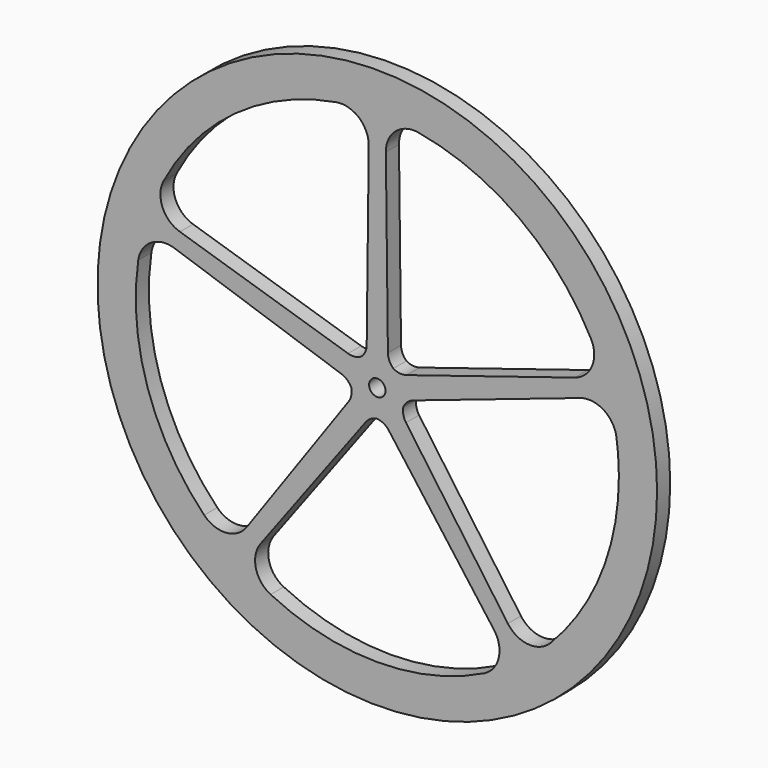
from build123d import *

# Parameters (mm, degrees)
F0_R        = 51.2
F1_DEPTH    = 1.5
F2_T1_DEPTH = 3
F3_R        = 5.08


# Not quite as in the source:
# - a fillet or chamfer that OpenCascade refuses, or shapes differently, is made with other operations: its cross-section is extruded or revolved along the edge and cut away or added


with BuildPart() as f1:
    # F0 (on Front) → F1 (new body, symmetric)
    with BuildSketch(Plane.XZ):
        Circle(F0_R)
        with BuildLine():
            ThreePointArc((1.5, 44.1745401787), (25.9801081513, 35.7585511514), (41.5489587997, 15.0772684084))
            ThreePointArc((41.5489587997, 15.0772684084), (42.0366980202, 13.6585511514), (42.4760097829, 12.2240988595))
            ThreePointArc((42.4760097829, 12.2240988595), (43.7668803572, 6.1725346333), (44.2, 0))
            ThreePointArc((44.2, 0), (39.7173586616, -19.3951391062), (27.1786687354, -34.8562758448))
            ThreePointArc((27.1786687354, -34.8562758448), (25.9801081513, -35.7585511514), (24.7516177523, -36.6196316017))
            ThreePointArc((24.7516177523, -36.6196316017), (0, -44.2), (-24.7516177523, -36.6196316017))
            ThreePointArc((-24.7516177523, -36.6196316017), (-25.9801081513, -35.7585511514), (-27.1786687354, -34.8562758448))
            ThreePointArc((-27.1786687354, -34.8562758448), (-42.0366980202, -13.6585511514), (-42.4760097829, 12.2240988595))
            ThreePointArc((-42.4760097829, 12.2240988595), (-42.0366980202, 13.6585511514), (-41.5489587997, 15.0772684084))
            ThreePointArc((-41.5489587997, 15.0772684084), (-25.9801081513, 35.7585511514), (-1.5, 44.1745401787))
            ThreePointArc((-1.5, 44.1745401787), (0, 44.2), (1.5, 44.1745401787))
        make_face(mode=Mode.SUBTRACT)
        with BuildLine():
            Line((-24.7516177523, -36.6196316017), (-1.118469097, -4.8732973313))
            ThreePointArc((-1.118469097, -4.8732973313), (-2.9389262615, -4.0450849719), (-4.2891552241, -2.569659017))
            Line((-4.2891552241, -2.569659017), (-27.1786687354, -34.8562758448))
            ThreePointArc((-27.1786687354, -34.8562758448), (-25.9801081513, -35.7585511514), (-24.7516177523, -36.6196316017))
        make_face()
        with BuildLine():
            ThreePointArc((-4.9804071414, -0.4422043711), (-4.7552825815, 1.5450849719), (-3.7693128085, 3.2851607193))
            Line((-3.7693128085, 3.2851607193), (-41.5489587997, 15.0772684084))
            ThreePointArc((-41.5489587997, 15.0772684084), (-42.0366980202, 13.6585511514), (-42.4760097829, 12.2240988595))
            Line((-42.4760097829, 12.2240988595), (-4.9804071414, -0.4422043711))
        make_face()
        with BuildLine():
            ThreePointArc((-1.9595917942, 4.6), (0, 5), (1.9595917942, 4.6))
            Line((1.9595917942, 4.6), (1.5, 44.1745401787))
            ThreePointArc((1.5, 44.1745401787), (0, 44.2), (-1.5, 44.1745401787))
            Line((-1.5, 44.1745401787), (-1.9595917942, 4.6))
        make_face()
        with BuildLine():
            ThreePointArc((3.7693128085, 3.2851607193), (4.6822304537, 1.7540575757), (5, 0))
            ThreePointArc((5, 0), (4.9950993837, -0.2213191055), (4.9804071414, -0.4422043711))
            Line((4.9804071414, -0.4422043711), (42.4760097829, 12.2240988595))
            ThreePointArc((42.4760097829, 12.2240988595), (42.0366980202, 13.6585511514), (41.5489587997, 15.0772684084))
            Line((41.5489587997, 15.0772684084), (3.7693128085, 3.2851607193))
        make_face()
        with BuildLine():
            Line((27.1786687354, -34.8562758448), (4.2891552241, -2.569659017))
            ThreePointArc((4.2891552241, -2.569659017), (2.9389262615, -4.0450849719), (1.118469097, -4.8732973313))
            Line((1.118469097, -4.8732973313), (24.7516177523, -36.6196316017))
            ThreePointArc((24.7516177523, -36.6196316017), (25.9801081513, -35.7585511514), (27.1786687354, -34.8562758448))
        make_face()
        with BuildLine():
            ThreePointArc((4.9804071414, -0.4422043711), (4.9950993837, -0.2213191055), (5, 0))
            ThreePointArc((5, 0), (4.6822304537, 1.7540575757), (3.7693128085, 3.2851607193))
            ThreePointArc((3.7693128085, 3.2851607193), (2.9389262615, 4.0450849719), (1.9595917942, 4.6))
            ThreePointArc((1.9595917942, 4.6), (0, 5), (-1.9595917942, 4.6))
            ThreePointArc((-1.9595917942, 4.6), (-2.9389262615, 4.0450849719), (-3.7693128085, 3.2851607193))
            ThreePointArc((-3.7693128085, 3.2851607193), (-4.7552825815, 1.5450849719), (-4.9804071414, -0.4422043711))
            ThreePointArc((-4.9804071414, -0.4422043711), (-4.7552825815, -1.5450849719), (-4.2891552241, -2.569659017))
            ThreePointArc((-4.2891552241, -2.569659017), (-2.9389262615, -4.0450849719), (-1.118469097, -4.8732973313))
            ThreePointArc((-1.118469097, -4.8732973313), (0, -5), (1.118469097, -4.8732973313))
            ThreePointArc((1.118469097, -4.8732973313), (2.9389262615, -4.0450849719), (4.2891552241, -2.569659017))
            ThreePointArc((4.2891552241, -2.569659017), (4.7552825815, -1.5450849719), (4.9804071414, -0.4422043711))
        make_face()
        with BuildLine():
            ThreePointArc((0, 1.5), (1.0606601718, 1.0606601718), (1.5, 0))
            ThreePointArc((1.5, 0), (-1.0606601718, -1.0606601718), (0, 1.5))
        make_face(mode=Mode.SUBTRACT)
    extrude(amount=F1_DEPTH, both=True)

    # F2: fillet of radius 3 on 10 edges, made by hand

    # F2_s2 → F2_t1 (join)
    with BuildSketch(Plane.XZ.offset(-1.5)):
        with BuildLine():
            ThreePointArc((3.0875868977, 3.9327861815), (2.2498717307, 4.9648804635), (1.9403413197, 6.2576202799))
            Line((1.9403413197, 6.2576202799), (1.9595917942, 4.6))
            ThreePointArc((1.9595917942, 4.6), (2.5455444913, 4.303510572), (3.0875868977, 3.9327861815))
        make_face()
        with BuildLine():
            ThreePointArc((2.7861851021, 4.151767404), (4.0266333175, 3.6739876086), (5.351752101, 3.7790852667))
            Line((5.351752101, 3.7790852667), (3.7693128085, 3.2851607193))
            ThreePointArc((3.7693128085, 3.2851607193), (3.3062652647, 3.7508145781), (2.7861851021, 4.151767404))
        make_face()
        with BuildLine():
            ThreePointArc((-2.7861851021, 4.151767404), (-4.0266333175, 3.6739876086), (-5.351752101, 3.7790852667))
            Line((-5.351752101, 3.7790852667), (-3.7693128085, 3.2851607193))
            ThreePointArc((-3.7693128085, 3.2851607193), (-3.3062652647, 3.7508145781), (-2.7861851021, 4.151767404))
        make_face()
        with BuildLine():
            ThreePointArc((-3.0875868977, 3.9327861815), (-2.2498717307, 4.9648804635), (-1.9403413197, 6.2576202799))
            Line((-1.9403413197, 6.2576202799), (-1.9595917942, 4.6))
            ThreePointArc((-1.9595917942, 4.6), (-2.5455444913, 4.303510572), (-3.0875868977, 3.9327861815))
        make_face()
        with BuildLine():
            ThreePointArc((-4.6944187481, -1.7211718734), (-5.4171305174, -0.605522732), (-6.5509489863, 0.0883367549))
            Line((-6.5509489863, 0.0883367549), (-4.9804071414, -0.4422043711))
            ThreePointArc((-4.9804071414, -0.4422043711), (-4.8794982801, -1.0910987737), (-4.6944187481, -1.7211718734))
        make_face()
        with BuildLine():
            ThreePointArc((-4.8095439897, -1.3668528124), (-4.7384679811, -2.6942312472), (-5.2479060175, -3.9220171386))
            Line((-5.2479060175, -3.9220171386), (-4.2891552241, -2.569659017))
            ThreePointArc((-4.2891552241, -2.569659017), (-4.5889288007, -1.9853796772), (-4.8095439897, -1.3668528124))
        make_face()
        with BuildLine():
            ThreePointArc((4.6944187481, -1.7211718734), (5.4171305174, -0.605522732), (6.5509489863, 0.0883367549))
            Line((6.5509489863, 0.0883367549), (4.9804071414, -0.4422043711))
            ThreePointArc((4.9804071414, -0.4422043711), (4.8794982801, -1.0910987737), (4.6944187481, -1.7211718734))
        make_face()
        with BuildLine():
            ThreePointArc((4.8095439897, -1.3668528124), (4.7384679811, -2.6942312472), (5.2479060175, -3.9220171386))
            Line((5.2479060175, -3.9220171386), (4.2891552241, -2.569659017))
            ThreePointArc((4.2891552241, -2.569659017), (4.5889288007, -1.9853796772), (4.8095439897, -1.3668528124))
        make_face()
        with BuildLine():
            ThreePointArc((0.186276554, -4.9965288997), (-1.0980990506, -5.3391140929), (-2.1083678125, -6.2030251629))
            Line((-2.1083678125, -6.2030251629), (-1.118469097, -4.8732973313))
            ThreePointArc((-1.118469097, -4.8732973313), (-0.4701512939, -4.9778466992), (0.186276554, -4.9965288997))
        make_face()
        with BuildLine():
            ThreePointArc((2.1083678125, -6.2030251629), (1.0980990506, -5.3391140929), (-0.186276554, -4.9965288997))
            ThreePointArc((-0.186276554, -4.9965288997), (0.4701512939, -4.9778466992), (1.118469097, -4.8732973313))
            Line((1.118469097, -4.8732973313), (2.1083678125, -6.2030251629))
        make_face()
    extrude(amount=F2_T1_DEPTH)

    # F3
    f3_edges = [f1.edges().sort_by_distance(p)[0] for p in [
        (-42.47601, 0, 12.224099),
        (42.47601, 0, 12.224099),
        (-1.5, 0, 44.17454),
        (24.751618, 0, -36.619632),
        (27.178669, 0, -34.856276),
        (41.548959, 0, 15.077268),
        (1.5, 0, 44.17454),
        (-41.548959, 0, 15.077268),
        (-27.178669, 0, -34.856276),
        (-24.751618, 0, -36.619632),
    ]]
    fillet(f3_edges, radius=F3_R)


solid = f1.part
